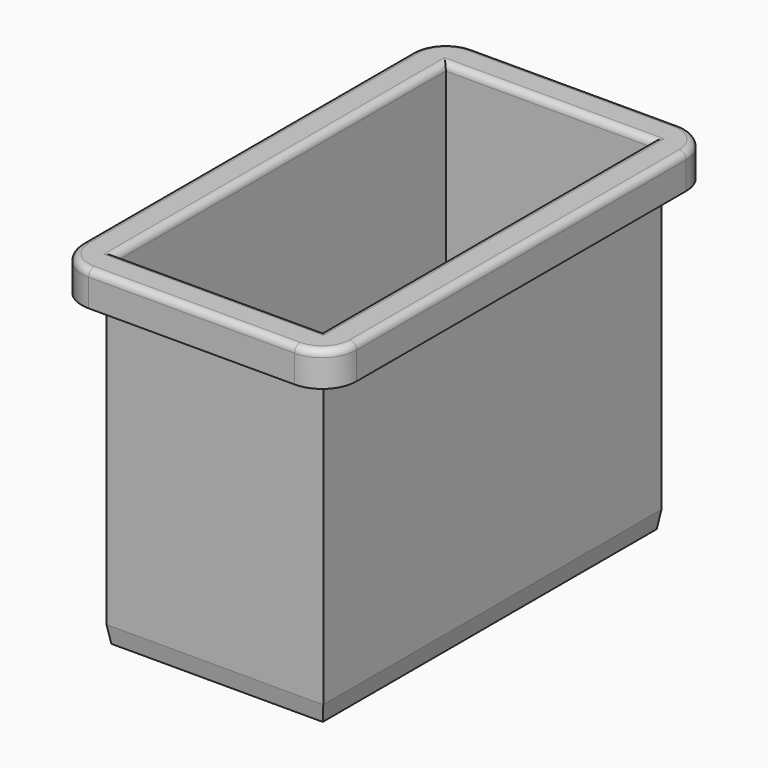
from build123d import *

# Parameters (mm, degrees)
F0_W     = 40.1
F0_H     = 78.2
F0_W_2   = 38.1
F0_H_2   = 76.2
F1_DEPTH = 6.35
F2_W     = 40.1
F2_H     = 78.2
F2_W_2   = 38.1
F2_H_2   = 76.2
F3_DEPTH = 57.15
F4_SIZE2 = 3.17499
F4_SIZE  = 0.49999
F5_R     = 1.27


# Not quite as in the source:
# - a fillet or chamfer is up to 0.001 mm smaller than in the source, because OpenCascade refuses the exact size


with BuildPart() as f1:
    # F0 (on Top) → F1 (new body)
    with BuildSketch(Plane.XY):
        with BuildLine():
            ThreePointArc((25.4, 38.1), (23.5401280605, 42.5901280605), (19.05, 44.45))
            Line((19.05, 44.45), (-19.05, 44.45))
            ThreePointArc((-19.05, 44.45), (-23.5401280605, 42.5901280605), (-25.4, 38.1))
            Line((-25.4, 38.1), (-25.4, -38.1))
            ThreePointArc((-25.4, -38.1), (-23.5401280605, -42.5901280605), (-19.05, -44.45))
            Line((-19.05, -44.45), (19.05, -44.45))
            ThreePointArc((19.05, -44.45), (23.5401280605, -42.5901280605), (25.4, -38.1))
            Line((25.4, -38.1), (25.4, 38.1))
        make_face()
        Rectangle(F0_W, F0_H, mode=Mode.SUBTRACT)
        Rectangle(F0_W, F0_H)
        Rectangle(F0_W_2, F0_H_2, mode=Mode.SUBTRACT)
    extrude(amount=F1_DEPTH)

    # F2 (on face) → F3 (join)
    with BuildSketch(Plane(origin=(0, 0, 0), x_dir=(1, 0, 0), z_dir=(0, 0, -1))):
        Rectangle(F2_W, F2_H)
        Rectangle(F2_W_2, F2_H_2, mode=Mode.SUBTRACT)
    extrude(amount=F3_DEPTH)

    # F4 (size 0.5 and 3.175 in the source; OpenCascade refuses exactly that, so slightly less here)
    f4_edges = [f1.edges().sort_by_distance(p)[0] for p in [
        (-20.05, 0, -57.15),
        (0, 39.1, -57.15),
        (20.05, 0, -57.15),
        (0, -39.1, -57.15),
        (0, -38.1, -57.15),
        (19.05, 0, -57.15),
        (0, 38.1, -57.15),
        (-19.05, 0, -57.15),
    ]]
    f4_side = f1.faces().sort_by_distance((-19.17118, 0, -57.15))[0]
    chamfer(f4_edges, length=F4_SIZE, length2=F4_SIZE2, reference=f4_side)

    # F5
    f5_edges = [f1.edges().sort_by_distance(p)[0] for p in [
        (23.540128, 42.590128, 6.35),
        (0, 44.45, 6.35),
        (-23.540128, 42.590128, 6.35),
        (-25.4, 0, 6.35),
        (-23.540128, -42.590128, 6.35),
        (0, -44.45, 6.35),
        (23.540128, -42.590128, 6.35),
        (25.4, 0, 6.35),
        (0, -38.1, 6.35),
        (-19.05, 0, 6.35),
        (0, 38.1, 6.35),
        (19.05, 0, 6.35),
    ]]
    fillet(f5_edges, radius=F5_R)


solid = f1.part
